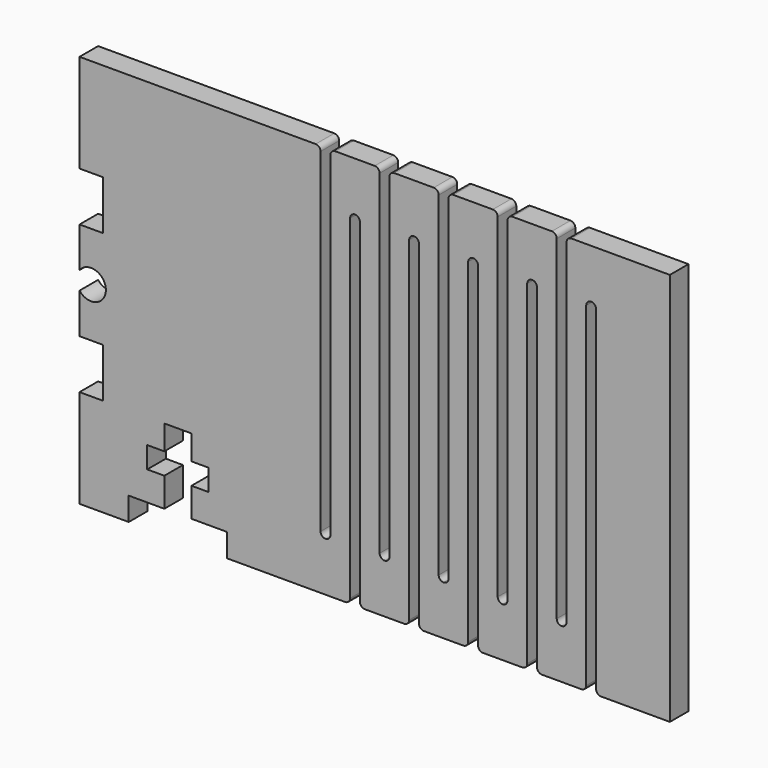
from build123d import *

# Parameters (mm, degrees)
F1_DEPTH = 3
F3_D     = 3.7973
F4_W     = 1.27
F4_H     = 44.4500002354
F4_H_2   = 44.45
F5_DEPTH = 3.001
F6_R     = 0.63499


# Not quite as in the source:
# - a fillet or chamfer is up to 0.001 mm smaller than in the source, because OpenCascade refuses the exact size


with BuildPart() as f1:
    # F0 (on Front) → F1 (new body)
    with BuildSketch(Plane.XZ):
        Polygon((38.1, 25.4), (-38.1, 25.4), (-38.1, 12.7), (-35.1, 12.7), (-35.1, 6.35), (-38.1, 6.35), (-38.1, -6.35), (-35.1, -6.35), (-35.1, -12.7), (-38.1, -12.7), (-38.1, -25.4), (-31.75, -25.4), (-31.75, -22.4), (-27.1526, -22.4), (-27.1526, -18.6436), (-29.3624, -18.6436), (-29.3624, -15.875), (-27.1526, -15.875), (-27.1526, -12.7), (-23.6474, -12.7), (-23.6474, -15.875), (-21.4376, -15.875), (-21.4376, -18.6436), (-23.6474, -18.6436), (-23.6474, -22.4), (-19.05, -22.4), (-19.05, -25.4), (38.1, -25.4), align=None)
    extrude(amount=F1_DEPTH)

    # F3 (through all)
    with Locations(Plane.XZ.offset(3)):
        with Locations((-36.6, 0)):
            Hole(F3_D / 2)

    # F4 (on face) → F5 (cut, through all)
    with BuildSketch(Plane.XZ.offset(3)):
        with Locations((-6.3499999233, 3.1749998823)):
            Rectangle(F4_W, F4_H)
        with Locations((-2.5399999233, -3.175)):
            Rectangle(F4_W, F4_H_2)
        with Locations((5.0800000767, -3.175)):
            Rectangle(F4_W, F4_H_2)
        with Locations((1.2700000767, 3.1749998823)):
            Rectangle(F4_W, F4_H)
        with Locations((12.7000000767, -3.175)):
            Rectangle(F4_W, F4_H_2)
        with Locations((8.8900000767, 3.1749998823)):
            Rectangle(F4_W, F4_H)
        with Locations((20.3200000767, -3.175)):
            Rectangle(F4_W, F4_H_2)
        with Locations((16.5100000767, 3.1749998823)):
            Rectangle(F4_W, F4_H)
        with Locations((27.9400000767, -3.175)):
            Rectangle(F4_W, F4_H_2)
        with Locations((24.1300000767, 3.1749998823)):
            Rectangle(F4_W, F4_H)
    extrude(amount=-F5_DEPTH, mode=Mode.SUBTRACT)

    # F6 (radius 0.635 in the source; OpenCascade refuses exactly that, so slightly less here)
    f6_edges = [f1.edges().sort_by_distance(p)[0] for p in [
        (-6.985, -1.5, -19.05),
        (-5.715, -1.5, -19.05),
        (0.635, -1.5, -19.05),
        (1.905, -1.5, -19.05),
        (9.525, -1.5, -19.05),
        (8.255, -1.5, -19.05),
        (15.875, -1.5, -19.05),
        (17.145, -1.5, -19.05),
        (24.765, -1.5, -19.05),
        (23.495, -1.5, -19.05),
        (-3.175, -1.5, 19.05),
        (4.445, -1.5, 19.05),
        (12.065, -1.5, 19.05),
        (19.685, -1.5, 19.05),
        (27.305, -1.5, 19.05),
        (-1.905, -1.5, 19.05),
        (5.715, -1.5, 19.05),
        (13.335, -1.5, 19.05),
        (20.955, -1.5, 19.05),
        (28.575, -1.5, 19.05),
        (-1.905, -1.5, -25.4),
        (4.445, -1.5, -25.4),
        (5.715, -1.5, -25.4),
        (12.065, -1.5, -25.4),
        (13.335, -1.5, -25.4),
        (19.685, -1.5, -25.4),
        (20.955, -1.5, -25.4),
        (27.305, -1.5, -25.4),
        (28.575, -1.5, -25.4),
        (-6.985, -1.5, 25.4),
        (-5.715, -1.5, 25.4),
        (-3.175, -1.5, -25.4),
        (0.635, -1.5, 25.4),
        (1.905, -1.5, 25.4),
        (8.255, -1.5, 25.4),
        (9.525, -1.5, 25.4),
        (15.875, -1.5, 25.4),
        (17.145, -1.5, 25.4),
        (23.495, -1.5, 25.4),
        (24.765, -1.5, 25.4),
    ]]
    fillet(f6_edges, radius=F6_R)


solid = f1.part
